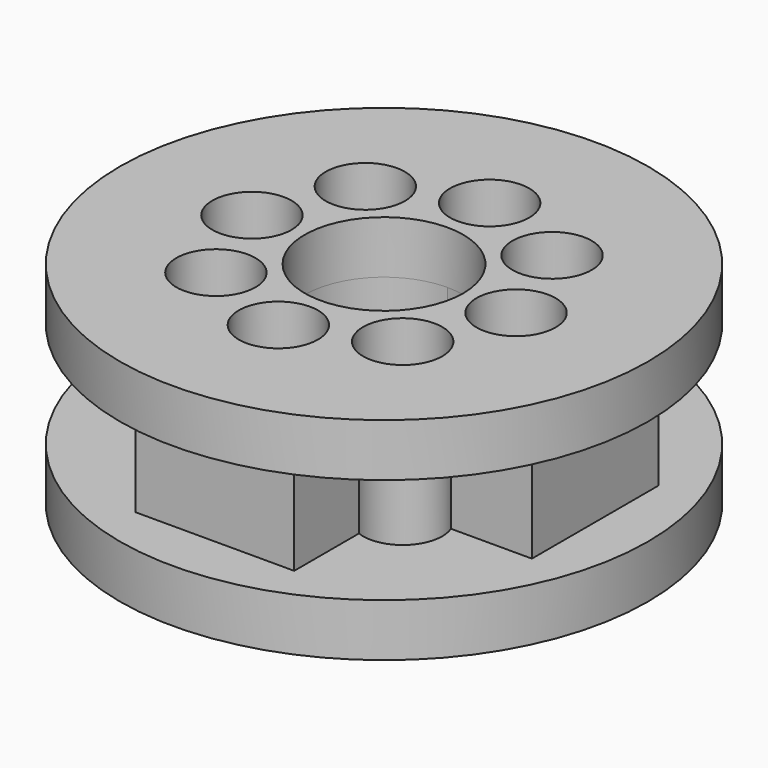
from build123d import *

# Parameters (mm, degrees)
F0_R     = 15.875
F0_R_2   = 4.7625
F1_DEPTH = 3.175
F3_DEPTH = 6.35
F4_R     = 15.875
F4_R_2   = 4.7625
F5_DEPTH = 3.175
F6_R     = 2.38125
F7_DEPTH = 25.4


with BuildPart() as f1:
    # F0 (on Top) → F1 (new body)
    with BuildSketch(Plane.XY):
        Circle(F0_R)
        Circle(F0_R_2, mode=Mode.SUBTRACT)
    extrude(amount=F1_DEPTH)

    # F2 (on face) → F3 (join)
    with BuildSketch(Plane.XY.offset(3.175)):
        with BuildLine():
            Line((4.7625, -4.7625), (4.7625, 0))
            ThreePointArc((4.7625, 0), (3.367596, -3.367596), (0, -4.7625))
            Line((0, -4.7625), (4.7625, -4.7625))
        make_face()
        with BuildLine():
            ThreePointArc((0, 4.7625), (3.367596, 3.367596), (4.7625, 0))
            Line((4.7625, 0), (4.7625, 4.7625))
            Line((4.7625, 4.7625), (0, 4.7625))
        make_face()
        Polygon((4.7625, 4.7625), (4.7625, 0), (4.7625, -4.7625), (12.7, -4.7625), (12.7, 4.7625), align=None)
        with BuildLine():
            ThreePointArc((-4.7625, 0), (-3.367596, 3.367596), (0, 4.7625))
            Line((0, 4.7625), (-4.7625, 4.7625))
            Line((-4.7625, 4.7625), (-4.7625, 0))
        make_face()
        Polygon((-4.7625, 4.7625), (0, 4.7625), (4.7625, 4.7625), (4.7625, 12.7), (-4.7625, 12.7), align=None)
        with BuildLine():
            Line((-4.7625, -4.7625), (0, -4.7625))
            ThreePointArc((0, -4.7625), (-3.367596, -3.367596), (-4.7625, 0))
            Line((-4.7625, 0), (-4.7625, -4.7625))
        make_face()
        Polygon((4.7625, -4.7625), (0, -4.7625), (-4.7625, -4.7625), (-4.7625, -12.7), (4.7625, -12.7), align=None)
        Polygon((-4.7625, -4.7625), (-4.7625, 0), (-4.7625, 4.7625), (-12.7, 4.7625), (-12.7, -4.7625), align=None)
    extrude(amount=F3_DEPTH)

    # F4 (on face) → F5 (join)
    with BuildSketch(Plane.XY.offset(9.525)):
        Circle(F4_R)
        Circle(F4_R_2, mode=Mode.SUBTRACT)
    extrude(amount=F5_DEPTH)

    # F6 (on face) → F7 (cut)
    with BuildSketch(Plane.XY.offset(12.7)):
        with Locations((-5.61266, 5.61266)):
            Circle(F6_R)
        with Locations((0, 7.9375)):
            Circle(F6_R)
        with Locations((5.61266, 5.61266)):
            Circle(F6_R)
        with Locations((7.9375, 0)):
            Circle(F6_R)
        with Locations((5.61266, -5.61266)):
            Circle(F6_R)
        with Locations((0, -7.9375)):
            Circle(F6_R)
        with Locations((-5.61266, -5.61266)):
            Circle(F6_R)
        with Locations((-7.9375, 0)):
            Circle(F6_R)
    extrude(amount=-F7_DEPTH, mode=Mode.SUBTRACT)


solid = f1.part
